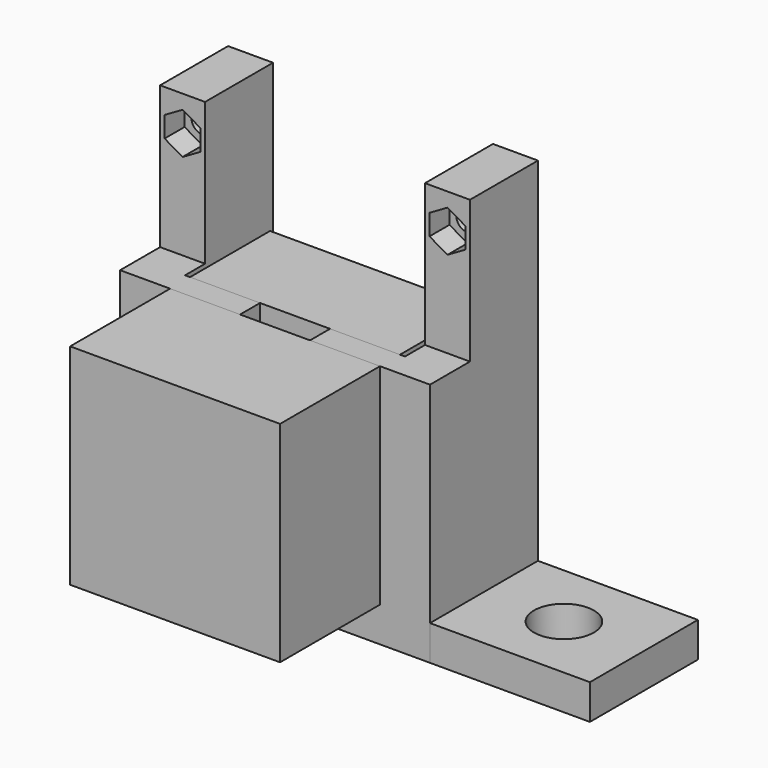
from build123d import *

# Parameters (mm, degrees)
F1_R      = 2.25
F2_DEPTH  = 12
F4_DEPTH  = 5
F5_W      = 44
F5_H      = 5
F6_DEPTH  = 7
F7_DEPTH  = 42
F8_R      = 1.7
F8_R_2    = 13
F9_DEPTH  = 5
F11_REACH = 63.8670687473
F12_R     = 1.7
F13_DEPTH = 20
F14_W     = 42
F14_H     = 42
F14_R     = 1.7
F14_R_2   = 13
F15_DEPTH = 25
F16_W     = 32
F16_H     = 27
F16_R     = 5.9941661127
F17_DEPTH = 7


with BuildPart() as f2:
    # F1 (on Front) → F2 (new body)
    with BuildSketch(Plane.XZ):
        Polygon((-27, 56.5), (-36, 56.5), (-36, -21), (26, -21), (26, 56.5), (17, 56.5), (17, -14), (-27, -14), align=None)
        with Locations((-31.5, 49.5)):
            Circle(F1_R, mode=Mode.SUBTRACT)
        with Locations((21.5, 49.5)):
            Circle(F1_R, mode=Mode.SUBTRACT)
    extrude(amount=-F2_DEPTH)

    # F3 (on face) → F4 (join)
    with BuildSketch(Plane.XZ):
        Polygon((-27, -14), (-27, 56.5), (-36, 56.5), (-36, -21), (26, -21), (26, 56.5), (17, 56.5), (17, -14), align=None)
        Polygon((-31.5, 53.6569219382), (-27.9, 51.5784609691), (-27.9, 47.4215390309), (-31.5, 45.3430780618), (-35.1, 47.4215390309), (-35.1, 51.5784609691), align=None, mode=Mode.SUBTRACT)
        Polygon((21.5, 53.6569219382), (25.1, 51.5784609691), (25.1, 47.4215390309), (21.5, 45.3430780618), (17.9, 47.4215390309), (17.9, 51.5784609691), align=None, mode=Mode.SUBTRACT)
    extrude(amount=F4_DEPTH)

    # F5 (on face) → F6 (join, through all)
    with BuildSketch(Plane.XY.offset(-14)):
        with Locations((-5, -7.5)):
            Rectangle(F5_W, F5_H)
        with Locations((-5, -12.5)):
            Rectangle(F5_W, F5_H)
        Polygon((-27, -10), (-27, -5), (-36, -5), (-36, -15), (-27, -15), align=None)
        Polygon((26, -5), (17, -5), (17, -10), (17, -15), (26, -15), align=None)
    extrude(amount=-F6_DEPTH)

    # F5 (on face) → F7 (join)
    with BuildSketch(Plane.XY.offset(-14)):
        with Locations((-5, -12.5)):
            Rectangle(F5_W, F5_H)
        Polygon((-27, -10), (-27, -5), (-36, -5), (-36, -15), (-27, -15), align=None)
        Polygon((26, -5), (17, -5), (17, -10), (17, -15), (26, -15), align=None)
    extrude(amount=F7_DEPTH)

    # F8 (on face) → F9 (cut, through all)
    with BuildSketch(Plane.XZ.offset(15)):
        with Locations((-20.5, 22.5)):
            Circle(F8_R)
        with Locations((-5, 7)):
            Circle(F8_R_2)
        with Locations((-20.5, -8.5)):
            Circle(F8_R)
        with Locations((10.5, -8.5)):
            Circle(F8_R)
        with Locations((10.5, 22.5)):
            Circle(F8_R)
    extrude(amount=-F9_DEPTH, mode=Mode.SUBTRACT)

    f11_end = f2.faces().sort_by_distance((-18, -12.5, 7))[0]
    # F10 (on face) → F11 (cut, up to a face of the model that its end follows)
    with BuildSketch(Plane.XY.offset(28)):
        Polygon((2, -10), (-5, -10), (-12, -10), (-12, -15), (2, -15), align=None)
    f11_long = extrude(amount=-F11_REACH, mode=Mode.PRIVATE)
    add(split(f11_long, bisect_by=f11_end, keep=Keep.ALL, mode=Mode.PRIVATE).solids().sort_by_distance((-5, -12.5, 28))[0], mode=Mode.SUBTRACT)


with BuildPart() as f13:
    # F12 (on face) → F13 (new body)
    with BuildSketch(Plane(origin=(0, -10, 0), x_dir=(-1, 0, 0), z_dir=(0, 1, 0))):
        with BuildLine():
            Line((-16, -14), (26, -14))
            Line((26, -14), (26, 28))
            Line((26, 28), (12, 28))
            Line((12, 28), (12, 17.9544511501))
            ThreePointArc((12, 17.9544511501), (5, -6), (-2, 17.9544511501))
            Line((-2, 17.9544511501), (-2, 28))
            Line((-2, 28), (-16, 28))
            Line((-16, 28), (-16, -14))
        make_face()
        with Locations((-10.5, -8.5)):
            Circle(F12_R, mode=Mode.SUBTRACT)
        with Locations((20.5, -8.5)):
            Circle(F12_R, mode=Mode.SUBTRACT)
        with Locations((-10.5, 22.5)):
            Circle(F12_R, mode=Mode.SUBTRACT)
        with Locations((20.5, 22.5)):
            Circle(F12_R, mode=Mode.SUBTRACT)
        with BuildLine():
            Line((12, 17.9544511501), (12, 28))
            Line((12, 28), (-2, 28))
            Line((-2, 28), (-2, 17.9544511501))
            ThreePointArc((-2, 17.9544511501), (5, -6), (12, 17.9544511501))
        make_face()
        with Locations((-10.5, 22.5)):
            Circle(F12_R)
        with Locations((20.5, 22.5)):
            Circle(F12_R)
        with Locations((-10.5, -8.5)):
            Circle(F12_R)
        with Locations((20.5, -8.5)):
            Circle(F12_R)
    extrude(amount=F13_DEPTH)


with BuildPart() as f15:
    # F14 (on face) → F15 (new body)
    with BuildSketch(Plane.XZ.offset(15)):
        with Locations((-5, 7)):
            Rectangle(F14_W, F14_H)
        with Locations((-20.5, -8.5)):
            Circle(F14_R, mode=Mode.SUBTRACT)
        with Locations((10.5, -8.5)):
            Circle(F14_R, mode=Mode.SUBTRACT)
        with Locations((-20.5, 22.5)):
            Circle(F14_R, mode=Mode.SUBTRACT)
        with Locations((-5, 7)):
            Circle(F14_R_2, mode=Mode.SUBTRACT)
        with Locations((10.5, 22.5)):
            Circle(F14_R, mode=Mode.SUBTRACT)
    extrude(amount=F15_DEPTH)

    # F8 (on face) → F15, piece 2 (join)
    with BuildSketch(Plane.XZ.offset(15)):
        with Locations((-20.5, 22.5)):
            Circle(F8_R)
    extrude(amount=F15_DEPTH)

    # F8 (on face) → F15, piece 3 (join)
    with BuildSketch(Plane.XZ.offset(15)):
        with Locations((-5, 7)):
            Circle(F8_R_2)
    extrude(amount=F15_DEPTH)

    # F8 (on face) → F15, piece 4 (join)
    with BuildSketch(Plane.XZ.offset(15)):
        with Locations((-20.5, -8.5)):
            Circle(F8_R)
    extrude(amount=F15_DEPTH)

    # F8 (on face) → F15, piece 5 (join)
    with BuildSketch(Plane.XZ.offset(15)):
        with Locations((10.5, 22.5)):
            Circle(F8_R)
    extrude(amount=F15_DEPTH)

    # F8 (on face) → F15, piece 6 (join)
    with BuildSketch(Plane.XZ.offset(15)):
        with Locations((10.5, -8.5)):
            Circle(F8_R)
    extrude(amount=F15_DEPTH)


with BuildPart() as f17:
    # F16 (on face) → F17 (new body, through all)
    with BuildSketch(Plane(origin=(0, 0, -21), x_dir=(1, 0, 0), z_dir=(0, 0, -1))):
        with Locations((42, 1.5)):
            Rectangle(F16_W, F16_H)
        with Locations((42, 1.5)):
            Circle(F16_R, mode=Mode.SUBTRACT)
    extrude(amount=-F17_DEPTH)


solid = Compound([f2.part, f13.part, f15.part, f17.part])
